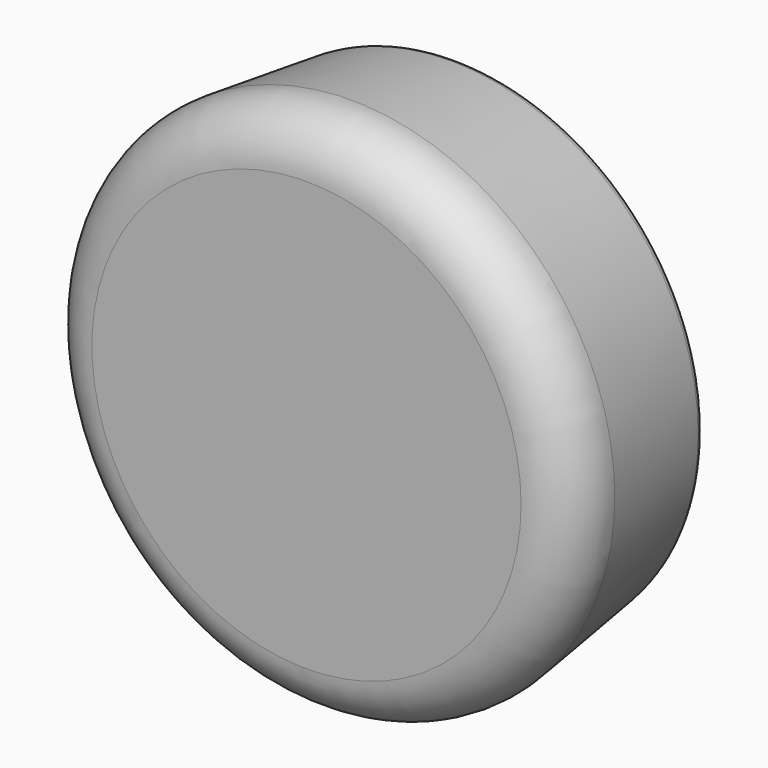
from build123d import *

# Parameters (mm, degrees)
F4_R  = 27.0285687642
F2_R  = 22.0858176649
F9_R  = 0.8852297765
F10_R = 4.9318127202


# Not quite as in the source:
# - the program builds the solid bodies; features that only make, move or delete a surface that nothing else refers to are left out


with BuildPart() as f5:
    # F4 (on offset) → F5 section 0
    with BuildSketch(Plane.XZ.offset(38.1)):
        Circle(F4_R)
    # F2 (on Front) → F5 section 1
    with BuildSketch(Plane.XZ):
        Circle(F2_R)
    loft()


with BuildPart() as f7:
    # F6 (on Front) → F7 (revolve)
    with BuildSketch(Plane.XZ):
        with BuildLine():
            ThreePointArc((0, -30.3672800573), (30.3672800573, 0), (0, 30.3672800573))
            Line((0, 30.3672800573), (0, -30.3672800573))
        make_face()
    revolve(axis=Axis((0, 0, 0), (0, 0, -1)))


with BuildPart() as f5_1:
    add(f5.part)

    # F8: cut F7
    add(f7.part, mode=Mode.SUBTRACT)

    # F9
    f9_edges = [f5_1.edges().sort_by_distance(p)[0] for p in [
        (-24.426448, -18.042182, 0),
    ]]
    fillet(f9_edges, radius=F9_R)

    # F10
    f10_edges = [f5_1.edges().sort_by_distance(p)[0] for p in [
        (-27.028569, -38.1, 0),
    ]]
    fillet(f10_edges, radius=F10_R)


solid = f5_1.part
